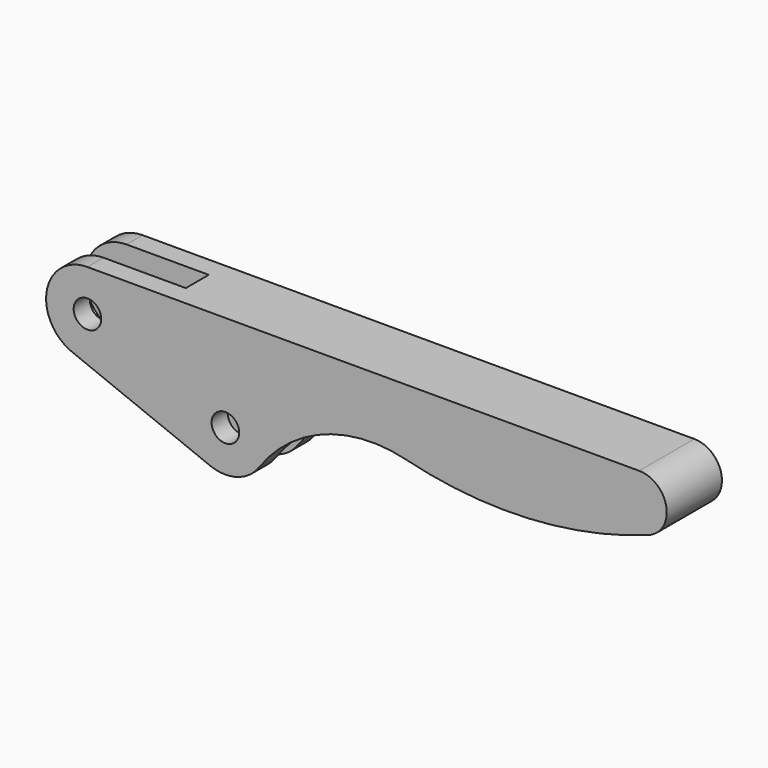
from build123d import *

# Parameters (mm, degrees)
F0_R     = 3.175
F1_DEPTH = 15.875
F2_W     = 76.2
F2_H     = 6.604
F3_DEPTH = 25.4


# Not quite as in the source:
# - a length typed as a fraction of an inch, garbled in the dataset ("3 / 203.2 mm" for 3/8 in), is restored


with BuildPart() as f1:
    # F0 (on Front) → F1 (new body)
    with BuildSketch(Plane.XZ):
        with BuildLine():
            Line((127, 9.525), (0, 9.525))
            ThreePointArc((0, 9.525), (-9.3531345836, 1.801249139), (-3.5374961923, -8.8437404807))
            Line((-3.5374961923, -8.8437404807), (28.2125038077, -21.5437404807))
            ThreePointArc((28.2125038077, -21.5437404807), (34.4639700258, -21.8301693138), (39.543916522, -18.1754442969))
            ThreePointArc((39.543916522, -18.1754442969), (54.4695569537, -6.6633605399), (73.291331011, -5.641775468))
            ThreePointArc((73.291331011, -5.641775468), (101.4455517982, -8.4127099235), (129.1718279101, -2.792048142))
            ThreePointArc((129.1718279101, -2.792048142), (133.2535292316, 4.2776659282), (127, 9.525))
        make_face()
        with Locations((31.75, -12.7)):
            Circle(F0_R, mode=Mode.SUBTRACT)
        Circle(F0_R, mode=Mode.SUBTRACT)
    extrude(amount=F1_DEPTH)

    # F2 (on face) → F3 (cut)
    with BuildSketch(Plane(origin=(-3.5374961923, 0, -8.8437404807), x_dir=(0.9284766909, 0, -0.3713906764), z_dir=(-0.3713906764, 0, -0.9284766909))):
        with Locations((17.0978982627, 7.9375)):
            Rectangle(F2_W, F2_H)
    extrude(amount=-F3_DEPTH, mode=Mode.SUBTRACT)


solid = f1.part
